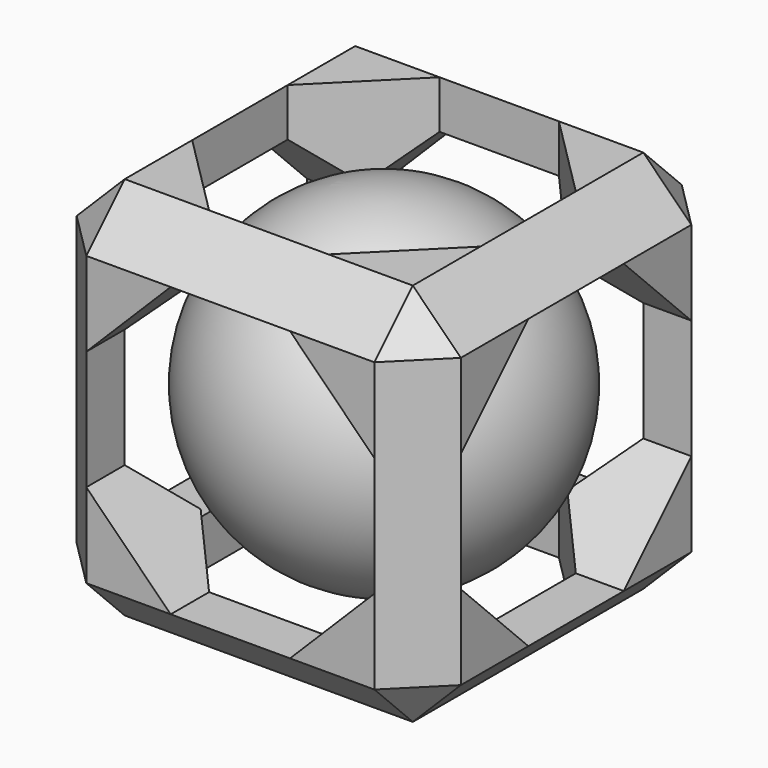
from build123d import *

# Parameters (mm, degrees)
F0_W     = 50.8
F0_H     = 50.8
F1_DEPTH = 50.8
F3_DEPTH = 50.801
F5_DEPTH = 50.801
F7_DEPTH = 50.801
F8_SIZE  = 6.34999


# Not quite as in the source:
# - a fillet or chamfer is up to 0.001 mm smaller than in the source, because OpenCascade refuses the exact size


with BuildPart() as f1:
    # F0 (on Top) → F1 (new body)
    with BuildSketch(Plane.XY):
        Rectangle(F0_W, F0_H)
    extrude(amount=F1_DEPTH)

    # F2 (on face) → F3 (cut, through all)
    with BuildSketch(Plane.XY.offset(50.8)):
        Polygon((7.8907683632, 19.05), (-7.8907683632, 19.05), (-19.05, 7.8907683632), (-19.05, -7.8907683632), (-7.8907683632, -19.05), (7.8907683632, -19.05), (19.05, -7.8907683632), (19.05, 7.8907683632), align=None)
    extrude(amount=-F3_DEPTH, mode=Mode.SUBTRACT)

    # F4 (on face) → F5 (cut, through all)
    with BuildSketch(Plane(origin=(-25.4, 0, 0), x_dir=(0, -1, 0), z_dir=(-1, 0, 0))):
        Polygon((-7.8907683632, 6.35), (7.8907683632, 6.35), (19.05, 17.5092316368), (19.05, 33.2907683632), (7.8907683632, 44.45), (-7.8907683632, 44.45), (-19.05, 33.2907683632), (-19.05, 17.5092316368), align=None)
    extrude(amount=-F5_DEPTH, mode=Mode.SUBTRACT)

    # F6 (on face) → F7 (cut, through all)
    with BuildSketch(Plane.XZ.offset(25.4)):
        Polygon((-7.8907683632, 6.35), (7.8907683632, 6.35), (19.05, 17.5092316368), (19.05, 33.2907683632), (7.8907683632, 44.45), (-7.8907683632, 44.45), (-19.05, 33.2907683632), (-19.05, 17.5092316368), align=None)
    extrude(amount=-F7_DEPTH, mode=Mode.SUBTRACT)

    # F8 (size 6.35 in the source; OpenCascade refuses exactly that, so slightly less here)
    f8_edges = [f1.edges().sort_by_distance(p)[0] for p in [
        (25.4, 0, 0),
        (0, -25.4, 0),
        (25.4, -25.4, 25.4),
        (25.4, 25.4, 25.4),
        (25.4, 0, 50.8),
        (0, 25.4, 50.8),
        (-25.4, 25.4, 25.4),
        (0, 25.4, 0),
        (-25.4, 0, 0),
        (-25.4, -25.4, 25.4),
        (-25.4, 0, 50.8),
        (0, -25.4, 50.8),
    ]]
    chamfer(f8_edges, length=F8_SIZE)


with BuildPart() as f11:
    # F9 (on Front) → F11 (revolve)
    with BuildSketch(Plane.XZ):
        with BuildLine():
            Line((0, 3.175), (0, 47.625))
            ThreePointArc((0, 47.625), (-22.225, 25.4), (0, 3.175))
        make_face()
    revolve(axis=Axis((0, 0, 27.8375800699), (0, 0, 1)))


solid = Compound([f1.part, f11.part])
